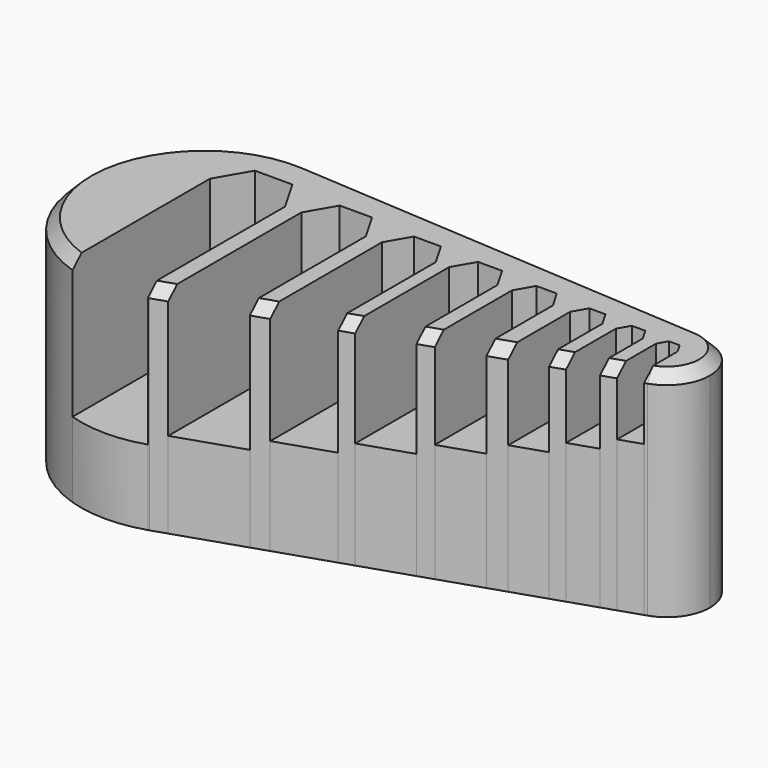
from build123d import *

# Parameters (mm, degrees)
F1_DEPTH       = 20
F2_DEPTH       = 14
F3_DEPTH       = 13
F4_DEPTH       = 12
F5_DEPTH       = 11
F6_DEPTH       = 10
F7_DEPTH       = 9
F8_DEPTH       = 8
F9_DEPTH       = 7
F10_T1_DEPTH   = 6.723420565
F10_T3_DEPTH   = 6.4600781335
F10_T5_DEPTH   = 6.5654151061
F10_T7_DEPTH   = 6.8287575376
F10_T9_DEPTH   = 6.4600781335
F10_T11_DEPTH  = 6.4600781335
F10_T13_DEPTH  = 4.0315664401
F10_T15_DEPTH  = 38.5986158262
F10_T17_DEPTH  = 2.842475063
F10_T20_ANGLE  = 178.7866538195
F10_T24_DEPTH  = 8.6433659759
F10_T30_DEPTH  = 8.6433659759
F10_T36_DEPTH  = 8.6433659759
F10_T42_DEPTH  = 8.1433659759
F10_T48_DEPTH  = 8.1433659759
F10_T54_DEPTH  = 8.1433659759
F10_T60_DEPTH  = 7.6433659759
F10_T66_DEPTH  = 7.6433659759
F10_T72_DEPTH  = 7.6433659759
F10_T78_DEPTH  = 7.3933659759
F10_T84_DEPTH  = 7.3933659759
F10_T90_DEPTH  = 7.3933659759
F10_T96_DEPTH  = 7.0433659759
F10_T102_DEPTH = 7.0433659759
F10_T108_DEPTH = 7.0433659759
F10_T114_DEPTH = 6.6433659759
F10_T120_DEPTH = 6.6433659759
F10_T126_DEPTH = 6.6433659759
F10_T130_ANGLE = 13.4104469015
F10_T132_ANGLE = 158.0080412786
F10_T137_DEPTH = 8.6433659759
F10_T141_DEPTH = 8.6433659759
F10_T149_DEPTH = 8.6433659759
F10_T153_DEPTH = 8.6433659759
F10_T161_DEPTH = 8.1433659759
F10_T166_DEPTH = 8.1433659759
F10_T173_DEPTH = 8.1433659759
F10_T177_DEPTH = 8.1433659759
F10_T185_DEPTH = 7.6433659759
F10_T190_DEPTH = 7.6433659759
F10_T197_DEPTH = 7.6433659759
F10_T201_DEPTH = 7.6433659759
F10_T209_DEPTH = 7.3933659759
F10_T214_DEPTH = 7.3933659759
F10_T221_DEPTH = 7.3933659759
F10_T226_DEPTH = 7.3933659759
F10_T233_DEPTH = 7.0433659759
F10_T238_DEPTH = 7.0433659759
F10_T246_DEPTH = 7.0433659759
F10_T251_DEPTH = 7.0433659759
F10_T259_DEPTH = 6.6433659759
F10_T264_DEPTH = 6.6433659759
F10_T272_DEPTH = 6.6433659759
F10_T277_DEPTH = 6.6433659759
F11_SIZE       = 0.5


# Not quite as in the source:
# - a fillet or chamfer that OpenCascade refuses, or shapes differently, is made with other operations: its cross-section is extruded or revolved along the edge and cut away or added


with BuildPart() as f1:
    # F0 (on Top) → F1 (new body)
    with BuildSketch(Plane.XY):
        with BuildLine():
            ThreePointArc((-17.3859174192, -15.9276489395), (-16.683828396, -15.6696039674), (-16, -15.3664622036))
            Line((-16, -15.3664622036), (-16, 0))
            Line((-16, 0), (-14.5, 2.5980762114))
            Line((-14.5, 2.5980762114), (-12.3766282, 2.5980762114))
            ThreePointArc((-12.3766282, 2.5980762114), (-15.9358837519, 5.3146518801), (-20.2628204012, 6.4660435079))
            ThreePointArc((-20.2628204012, 6.4660435079), (-32.3001541206, -2.8757046875), (-24.5, -15.9647557651))
            Line((-24.5, -15.9647557651), (-24.5, 0))
            Line((-24.5, 0), (-22.75, 3.0310889132))
            Line((-22.75, 3.0310889132), (-19.25, 3.0310889132))
            Line((-19.25, 3.0310889132), (-17.5, 0))
            Line((-17.5, 0), (-17.5, -15.9647557651))
            ThreePointArc((-17.5, -15.9647557651), (-17.4429103229, -15.9463511141), (-17.3859174192, -15.9276489395))
        make_face()
        with BuildLine():
            Line((-2.25, 0), (-1.125, 1.9485571585))
            Line((-1.125, 1.9485571585), (1.125, 1.9485571585))
            Line((1.125, 1.9485571585), (2.25, 0))
            Line((2.25, 0), (2.25, -9.4273659957))
            Line((2.25, -9.4273659957), (3.6, -8.9804613879))
            Line((3.6, -8.9804613879), (3.6, 0))
            Line((3.6, 0), (4.55, 1.6454482672))
            Line((4.55, 1.6454482672), (6.45, 1.6454482672))
            Line((6.45, 1.6454482672), (7.4, 0))
            Line((7.4, 0), (7.4, -7.7225076769))
            Line((7.4, -7.7225076769), (9, -7.1928429565))
            Line((9, -7.1928429565), (9, 0))
            Line((9, 0), (9.75, 1.2990381057))
            Line((9.75, 1.2990381057), (11.25, 1.2990381057))
            Line((11.25, 1.2990381057), (12, 0))
            Line((12, 0), (12, -6.1997216057))
            Line((12, -6.1997216057), (13.25, -5.7859210429))
            Line((13.25, -5.7859210429), (13.25, 0))
            Line((13.25, 0), (13.875, 1.0825317547))
            Line((13.875, 1.0825317547), (14.1492695498, 1.0825317547))
            ThreePointArc((14.1492695498, 1.0825317547), (15.6879217246, 3.2640916115), (18.2564102564, 3.9917732627))
            Line((18.2564102564, 3.9917732627), (-20.2628204012, 6.4660435079))
            ThreePointArc((-20.2628204012, 6.4660435079), (-15.9358837519, 5.3146518801), (-12.3766282, 2.5980762114))
            Line((-12.3766282, 2.5980762114), (-11.5, 2.5980762114))
            Line((-11.5, 2.5980762114), (-10, 0))
            Line((-10, 0), (-10, -1.6562026488))
            ThreePointArc((-10, -1.6562026488), (-9.6256868339, -3.3147221192), (-9.5, -5.010304615))
            ThreePointArc((-9.5, -5.010304615), (-9.6256868339, -6.7058871108), (-10, -8.3644065813))
            Line((-10, -8.3644065813), (-10, -13.4826115115))
            Line((-10, -13.4826115115), (-8.5, -12.9860508361))
            Line((-8.5, -12.9860508361), (-8.5, 0))
            Line((-8.5, 0), (-7.25, 2.1650635095))
            Line((-7.25, 2.1650635095), (-4.75, 2.1650635095))
            Line((-4.75, 2.1650635095), (-3.5, 0))
            Line((-3.5, 0), (-3.5, -11.3308485847))
            Line((-3.5, -11.3308485847), (-2.25, -10.9170480219))
            Line((-2.25, -10.9170480219), (-2.25, 0))
        make_face()
        with BuildLine():
            Line((15.75, 0), (15.75, -3.3071891388))
            ThreePointArc((15.75, -3.3071891388), (16.3505589519, -3.6440834552), (17, -3.8729833462))
            Line((17, -3.8729833462), (17, 0))
            Line((17, 0), (17.5, 0.8660254038))
            Line((17.5, 0.8660254038), (18.5, 0.8660254038))
            Line((18.5, 0.8660254038), (19, 0))
            Line((19, 0), (19, -3.8729833462))
            ThreePointArc((19, -3.8729833462), (19.1291697471, -3.8373136023), (19.257072202, -3.7973371563))
            ThreePointArc((19.257072202, -3.7973371563), (21.2425521436, -2.3421903415), (22, 0))
            ThreePointArc((22, 0), (20.9176738188, 2.7362710917), (18.2564102564, 3.9917732627))
            ThreePointArc((18.2564102564, 3.9917732627), (15.6879217246, 3.2640916115), (14.1492695498, 1.0825317547))
            Line((14.1492695498, 1.0825317547), (15.125, 1.0825317547))
            Line((15.125, 1.0825317547), (15.75, 0))
        make_face()
        with BuildLine():
            Line((-10, -1.6562026488), (-10, -8.3644065813))
            ThreePointArc((-10, -8.3644065813), (-9.6256868339, -6.7058871108), (-9.5, -5.010304615))
            ThreePointArc((-9.5, -5.010304615), (-9.6256868339, -3.3147221192), (-10, -1.6562026488))
        make_face()
        with BuildLine():
            Line((15.75, -3.3071891388), (15.75, -4.9583199172))
            Line((15.75, -4.9583199172), (17, -4.5445193544))
            Line((17, -4.5445193544), (17, -3.8729833462))
            ThreePointArc((17, -3.8729833462), (16.3505589519, -3.6440834552), (15.75, -3.3071891388))
        make_face()
        with BuildLine():
            Line((19, -3.8729833462), (19, -3.8824384538))
            Line((19, -3.8824384538), (19.257072202, -3.7973371563))
            ThreePointArc((19.257072202, -3.7973371563), (19.1291697471, -3.8373136023), (19, -3.8729833462))
        make_face()
        with BuildLine():
            Line((-17.3859174192, -15.9276489395), (-16, -15.468854213))
            Line((-16, -15.468854213), (-16, -15.3664622036))
            ThreePointArc((-16, -15.3664622036), (-16.683828396, -15.6696039674), (-17.3859174192, -15.9276489395))
        make_face()
    extrude(amount=F1_DEPTH)

    # F0 (on Top) → F2 (join)
    with BuildSketch(Plane.XY):
        with BuildLine():
            Line((17, 0), (17, -3.8729833462))
            ThreePointArc((17, -3.8729833462), (18, -4), (19, -3.8729833462))
            Line((19, -3.8729833462), (19, 0))
            Line((19, 0), (18.5, -0.8660254038))
            Line((18.5, -0.8660254038), (17.5, -0.8660254038))
            Line((17.5, -0.8660254038), (17, 0))
        make_face()
        with BuildLine():
            Line((17, -3.8729833462), (17, -4.5445193544))
            Line((17, -4.5445193544), (19, -3.8824384538))
            Line((19, -3.8824384538), (19, -3.8729833462))
            ThreePointArc((19, -3.8729833462), (18, -4), (17, -3.8729833462))
        make_face()
    extrude(amount=F2_DEPTH)

    # F0 (on Top) → F3 (join)
    with BuildSketch(Plane.XY):
        with BuildLine():
            Line((13.25, 0), (13.25, -5.7859210429))
            Line((13.25, -5.7859210429), (15.75, -4.9583199172))
            Line((15.75, -4.9583199172), (15.75, -3.3071891388))
            ThreePointArc((15.75, -3.3071891388), (14.7531548966, -2.3362356205), (14.1492695498, -1.0825317547))
            Line((14.1492695498, -1.0825317547), (13.875, -1.0825317547))
            Line((13.875, -1.0825317547), (13.25, 0))
        make_face()
        with BuildLine():
            ThreePointArc((14.1492695498, -1.0825317547), (14.7531548966, -2.3362356205), (15.75, -3.3071891388))
            Line((15.75, -3.3071891388), (15.75, 0))
            Line((15.75, 0), (15.125, -1.0825317547))
            Line((15.125, -1.0825317547), (14.1492695498, -1.0825317547))
        make_face()
    extrude(amount=F3_DEPTH)

    # F0 (on Top) → F4 (join)
    with BuildSketch(Plane.XY):
        Polygon((9, 0), (9, -7.1928429565), (12, -6.1997216057), (12, 0), (11.25, -1.2990381057), (9.75, -1.2990381057), align=None)
    extrude(amount=F4_DEPTH)

    # F0 (on Top) → F5 (join)
    with BuildSketch(Plane.XY):
        Polygon((3.6, 0), (3.6, -8.9804613879), (7.4, -7.7225076769), (7.4, 0), (6.45, -1.6454482672), (4.55, -1.6454482672), align=None)
    extrude(amount=F5_DEPTH)

    # F0 (on Top) → F6 (join)
    with BuildSketch(Plane.XY):
        Polygon((-1.125, -1.9485571585), (-2.25, 0), (-2.25, -10.9170480219), (2.25, -9.4273659957), (2.25, 0), (1.125, -1.9485571585), align=None)
    extrude(amount=F6_DEPTH)

    # F0 (on Top) → F7 (join)
    with BuildSketch(Plane.XY):
        Polygon((-8.5, -12.9860508361), (-3.5, -11.3308485847), (-3.5, 0), (-4.75, -2.1650635095), (-7.25, -2.1650635095), (-8.5, 0), align=None)
    extrude(amount=F7_DEPTH)

    # F0 (on Top) → F8 (join)
    with BuildSketch(Plane.XY):
        with BuildLine():
            Line((-16, -15.468854213), (-10, -13.4826115115))
            Line((-10, -13.4826115115), (-10, -8.3644065813))
            ThreePointArc((-10, -8.3644065813), (-12.2674633849, -12.4931385879), (-16, -15.3664622036))
            Line((-16, -15.3664622036), (-16, -15.468854213))
        make_face()
        with BuildLine():
            ThreePointArc((-16, -15.3664622036), (-12.2674633849, -12.4931385879), (-10, -8.3644065813))
            Line((-10, -8.3644065813), (-10, -1.6562026488))
            ThreePointArc((-10, -1.6562026488), (-10.1707020381, -1.1403814048), (-10.3655774228, -0.6331986704))
            Line((-10.3655774228, -0.6331986704), (-11.5, -2.5980762114))
            Line((-11.5, -2.5980762114), (-14.5, -2.5980762114))
            Line((-14.5, -2.5980762114), (-16, 0))
            Line((-16, 0), (-16, -15.3664622036))
        make_face()
        with BuildLine():
            ThreePointArc((-10.3655774228, -0.6331986704), (-10.1707020381, -1.1403814048), (-10, -1.6562026488))
            Line((-10, -1.6562026488), (-10, 0))
            Line((-10, 0), (-10.3655774228, -0.6331986704))
        make_face()
    extrude(amount=F8_DEPTH)

    # F0 (on Top) → F9 (join)
    with BuildSketch(Plane.XY):
        with BuildLine():
            ThreePointArc((-24.5, -15.9647557651), (-21, -16.510304615), (-17.5, -15.9647557651))
            Line((-17.5, -15.9647557651), (-17.5, 0))
            Line((-17.5, 0), (-19.25, -3.0310889132))
            Line((-19.25, -3.0310889132), (-22.75, -3.0310889132))
            Line((-22.75, -3.0310889132), (-24.5, 0))
            Line((-24.5, 0), (-24.5, -15.9647557651))
        make_face()
    extrude(amount=F9_DEPTH)

    # F10: chamfer of 1 on 29 edges, made by hand

    # F10_s2 → F10_t1 (cut)
    with BuildSketch(Plane(origin=(-15.4762183794, -5.1232543007, 0), x_dir=(0, 0, 1), z_dir=(0.9493342891, 0.3142680505, 0))):
        Polygon((20, 8.6568249091), (19, 9.6568249091), (20, 9.6568249091), align=None)
    extrude(amount=F10_T1_DEPTH, mode=Mode.SUBTRACT)

    # F10_s4 → F10_t3 (cut)
    with BuildSketch(Plane(origin=(-8.9762183794, -2.971491374, 0), x_dir=(0, 0, 1), z_dir=(0.9493342891, 0.3142680505, 0))):
        Polygon((20, 8.6568249091), (19, 9.6568249091), (20, 9.6568249091), align=None)
    extrude(amount=F10_T3_DEPTH, mode=Mode.SUBTRACT)

    # F10_s6 → F10_t5 (cut)
    with BuildSketch(Plane(origin=(-3.2262183794, -1.068008785, 0), x_dir=(0, 0, 1), z_dir=(0.9493342891, 0.3142680505, 0))):
        Polygon((20, 8.6568249091), (19, 9.6568249091), (20, 9.6568249091), align=None)
    extrude(amount=F10_T5_DEPTH, mode=Mode.SUBTRACT)

    # F10_s8 → F10_t7 (cut)
    with BuildSketch(Plane(origin=(1.9237816206, 0.6368495339, 0), x_dir=(0, 0, 1), z_dir=(0.9493342891, 0.3142680505, 0))):
        Polygon((20, 8.6568249091), (19, 9.6568249091), (20, 9.6568249091), align=None)
    extrude(amount=F10_T7_DEPTH, mode=Mode.SUBTRACT)

    # F10_s10 → F10_t9 (cut)
    with BuildSketch(Plane(origin=(6.5237816206, 2.1596356051, 0), x_dir=(0, 0, 1), z_dir=(0.9493342891, 0.3142680505, 0))):
        Polygon((20, 8.6568249091), (19, 9.6568249091), (20, 9.6568249091), align=None)
    extrude(amount=F10_T9_DEPTH, mode=Mode.SUBTRACT)

    # F10_s12 → F10_t11 (cut)
    with BuildSketch(Plane(origin=(10.2737816206, 3.4010372936, 0), x_dir=(0, 0, 1), z_dir=(0.9493342891, 0.3142680505, 0))):
        Polygon((20, 8.6568249091), (19, 9.6568249091), (20, 9.6568249091), align=None)
    extrude(amount=F10_T11_DEPTH, mode=Mode.SUBTRACT)

    # F10_s14 → F10_t13 (cut)
    with BuildSketch(Plane(origin=(-20.4207489575, -6.7600939296, 0), x_dir=(0, 0, 1), z_dir=(0.9493342891, 0.3142680505, 0))):
        Polygon((20, 8.6568249091), (19, 9.6568249091), (20, 9.6568249091), align=None)
    extrude(amount=F10_T13_DEPTH, mode=Mode.SUBTRACT)

    # F10_s16 → F10_t15 (cut)
    with BuildSketch(Plane(origin=(17.926035503, -1.1514730565, 0), x_dir=(0, 0, 1), z_dir=(-0.9979433157, 0.0641025641, 0))):
        Polygon((20, 4.1538461538), (19, 5.1538461538), (20, 5.1538461538), align=None)
    extrude(amount=F10_T15_DEPTH, mode=Mode.SUBTRACT)

    # F10_s18 → F10_t17 (cut)
    with BuildSketch(Plane(origin=(13.5237816206, 4.4769187569, 0), x_dir=(0, 0, 1), z_dir=(0.9493342891, 0.3142680505, 0))):
        Polygon((20, 8.6568249091), (19, 9.6568249091), (20, 9.6568249091), align=None)
    extrude(amount=F10_T17_DEPTH, mode=Mode.SUBTRACT)

    # F10_s19 → F10_t20 (revolve, cut)
    with BuildSketch(Plane(origin=(-20.5931951918, 1.3227973923, 0), x_dir=(0, 0, 1), z_dir=(0.997943315, -0.0641025738, 0))):
        Polygon((20, -4.1538459531), (19, -5.1538459533), (20, -5.1538459531), align=None)
    revolve(axis=Axis((-21, -5.010304615, 20), (0, 0, 1)), revolution_arc=F10_T20_ANGLE, mode=Mode.SUBTRACT)


with BuildPart() as f10_tool22:
    # F10_s23 → F10_t24 (new body)
    with BuildSketch(Plane.YZ.offset(-16.678317012)):
        Polygon((-4.0310889132, 7), (-3.0310889132, 6), (-3.0310889132, 7), align=None)
    extrude(amount=-F10_T24_DEPTH)

    split(bisect_by=Plane(origin=(-18.375, -10.6088111964, 0), x_dir=(0, 0, 1), z_dir=(0.8660254038, 0.5, 0)), keep=Keep.TOP)

    split(bisect_by=Plane(origin=(-13.125, 7.5777222831, 0), x_dir=(0, 0, 1), z_dir=(-0.8660254038, 0.5, 0)), keep=Keep.TOP)


with BuildPart() as f1_1:
    add(f1.part)

    # F10_t21: cut F10_tool22
    add(f10_tool22.part, mode=Mode.SUBTRACT)


with BuildPart() as f10_tool28:
    # F10_s29 → F10_t30 (new body)
    with BuildSketch(Plane(origin=(-3.089158506, 5.3505794851, 0), x_dir=(0, 0, 1), z_dir=(-0.5, 0.8660254038, 0))):
        Polygon((6, -21.2176223927), (7, -22.2176223927), (7, -21.2176223927), align=None)
    extrude(amount=F10_T30_DEPTH)

    split(bisect_by=Plane.XZ.offset(3.0310889132), keep=Keep.BOTTOM)

    split(bisect_by=Plane.YZ.offset(-24.5), keep=Keep.TOP)


with BuildPart() as f1_2:
    add(f1_1.part)

    # F10_t27: cut F10_tool28
    add(f10_tool28.part, mode=Mode.SUBTRACT)


with BuildPart() as f10_tool34:
    # F10_s35 → F10_t36 (new body)
    with BuildSketch(Plane(origin=(-3.089158506, -5.3505794851, 0), x_dir=(0, 0, 1), z_dir=(-0.5, -0.8660254038, 0))):
        Polygon((7, 14.1554445662), (6, 15.1554445662), (7, 15.1554445662), align=None)
    extrude(amount=F10_T36_DEPTH)

    split(bisect_by=Plane.XZ.offset(3.0310889132), keep=Keep.BOTTOM)

    split(bisect_by=Plane.YZ.offset(-17.5), keep=Keep.BOTTOM)


with BuildPart() as f1_3:
    add(f1_2.part)

    # F10_t33: cut F10_tool34
    add(f10_tool34.part, mode=Mode.SUBTRACT)


with BuildPart() as f10_tool40:
    # F10_s41 → F10_t42 (new body)
    with BuildSketch(Plane(origin=(-1.214158506, 2.1029842209, 0), x_dir=(0, 0, 1), z_dir=(-0.5, 0.8660254038, 0))):
        Polygon((8, -14.8564064606), (7, -13.8564064606), (8, -13.8564064606), align=None)
    extrude(amount=F10_T42_DEPTH)

    split(bisect_by=Plane.XZ.offset(2.5980762114), keep=Keep.BOTTOM)

    split(bisect_by=Plane.YZ.offset(-16), keep=Keep.TOP)


with BuildPart() as f1_4:
    add(f1_3.part)

    # F10_t39: cut F10_tool40
    add(f10_tool40.part, mode=Mode.SUBTRACT)


with BuildPart() as f10_tool46:
    # F10_s47 → F10_t48 (new body)
    with BuildSketch(Plane.YZ.offset(-8.928317012)):
        Polygon((-3.5980762114, 8), (-2.5980762114, 7), (-2.5980762114, 8), align=None)
    extrude(amount=-F10_T48_DEPTH)

    split(bisect_by=Plane(origin=(-12, -6.9282032303, 0), x_dir=(0, 0, 1), z_dir=(0.8660254038, 0.5, 0)), keep=Keep.TOP)

    split(bisect_by=Plane(origin=(-7.5, 4.3301270189, 0), x_dir=(0, 0, 1), z_dir=(-0.8660254038, 0.5, 0)), keep=Keep.TOP)


with BuildPart() as f1_5:
    add(f1_4.part)

    # F10_t45: cut F10_tool46
    add(f10_tool46.part, mode=Mode.SUBTRACT)


with BuildPart() as f10_tool52:
    # F10_s53 → F10_t54 (new body)
    with BuildSketch(Plane(origin=(-1.214158506, -2.1029842209, 0), x_dir=(0, 0, 1), z_dir=(-0.5, -0.8660254038, 0))):
        Polygon((8, 7.6602540378), (7, 8.6602540378), (8, 8.6602540378), align=None)
    extrude(amount=F10_T54_DEPTH)

    split(bisect_by=Plane.YZ.offset(-10), keep=Keep.BOTTOM)

    split(bisect_by=Plane.XZ.offset(2.5980762114), keep=Keep.BOTTOM)


with BuildPart() as f1_6:
    add(f1_5.part)

    # F10_t51: cut F10_tool52
    add(f10_tool52.part, mode=Mode.SUBTRACT)


with BuildPart() as f10_tool58:
    # F10_s59 → F10_t60 (new body)
    with BuildSketch(Plane(origin=(0.410841494, -0.7115983414, 0), x_dir=(0, 0, 1), z_dir=(-0.5, 0.8660254038, 0))):
        Polygon((9, -8.3612159322), (8, -7.3612159322), (9, -7.3612159322), align=None)
    extrude(amount=F10_T60_DEPTH)

    split(bisect_by=Plane.XZ.offset(2.1650635095), keep=Keep.BOTTOM)

    split(bisect_by=Plane.YZ.offset(-8.5), keep=Keep.TOP)


with BuildPart() as f1_7:
    add(f1_6.part)

    # F10_t57: cut F10_tool58
    add(f10_tool58.part, mode=Mode.SUBTRACT)


with BuildPart() as f10_tool64:
    # F10_s65 → F10_t66 (new body)
    with BuildSketch(Plane.YZ.offset(-2.178317012)):
        Polygon((-3.1650635095, 9), (-2.1650635095, 8), (-2.1650635095, 9), align=None)
    extrude(amount=-F10_T66_DEPTH)

    split(bisect_by=Plane(origin=(-6.375, -3.6806079661, 0), x_dir=(0, 0, 1), z_dir=(0.8660254038, 0.5, 0)), keep=Keep.TOP)

    split(bisect_by=Plane(origin=(-2.625, 1.5155444566, 0), x_dir=(0, 0, 1), z_dir=(-0.8660254038, 0.5, 0)), keep=Keep.TOP)


with BuildPart() as f1_8:
    add(f1_7.part)

    # F10_t63: cut F10_tool64
    add(f10_tool64.part, mode=Mode.SUBTRACT)


with BuildPart() as f10_tool70:
    # F10_s71 → F10_t72 (new body)
    with BuildSketch(Plane(origin=(0.410841494, 0.7115983414, 0), x_dir=(0, 0, 1), z_dir=(-0.5, -0.8660254038, 0))):
        Polygon((9, 2.0310889132), (8, 3.0310889132), (9, 3.0310889132), align=None)
    extrude(amount=F10_T72_DEPTH)

    split(bisect_by=Plane.YZ.offset(-3.5), keep=Keep.BOTTOM)

    split(bisect_by=Plane.XZ.offset(2.1650635095), keep=Keep.BOTTOM)


with BuildPart() as f1_9:
    add(f1_8.part)

    # F10_t69: cut F10_tool70
    add(f10_tool70.part, mode=Mode.SUBTRACT)


with BuildPart() as f10_tool76:
    # F10_s77 → F10_t78 (new body)
    with BuildSketch(Plane(origin=(1.848341494, -3.2014213773, 0), x_dir=(0, 0, 1), z_dir=(-0.5, 0.8660254038, 0))):
        Polygon((10, -2.9485571585), (9, -1.9485571585), (10, -1.9485571585), align=None)
    extrude(amount=F10_T78_DEPTH)

    split(bisect_by=Plane.XZ.offset(1.9485571585), keep=Keep.BOTTOM)

    split(bisect_by=Plane.YZ.offset(-2.25), keep=Keep.TOP)


with BuildPart() as f1_10:
    add(f1_9.part)

    # F10_t75: cut F10_tool76
    add(f10_tool76.part, mode=Mode.SUBTRACT)


with BuildPart() as f10_tool82:
    # F10_s83 → F10_t84 (new body)
    with BuildSketch(Plane.YZ.offset(3.696682988)):
        Polygon((-2.9485571585, 10), (-1.9485571585, 9), (-1.9485571585, 10), align=None)
    extrude(amount=-F10_T84_DEPTH)

    split(bisect_by=Plane(origin=(1.6875, -0.9742785793, 0), x_dir=(0, 0, 1), z_dir=(-0.8660254038, 0.5, 0)), keep=Keep.TOP)

    split(bisect_by=Plane(origin=(-1.6875, -0.9742785793, 0), x_dir=(0, 0, 1), z_dir=(0.8660254038, 0.5, 0)), keep=Keep.TOP)


with BuildPart() as f1_11:
    add(f1_10.part)

    # F10_t81: cut F10_tool82
    add(f10_tool82.part, mode=Mode.SUBTRACT)


with BuildPart() as f10_tool88:
    # F10_s89 → F10_t90 (new body)
    with BuildSketch(Plane(origin=(1.848341494, 3.2014213773, 0), x_dir=(0, 0, 1), z_dir=(-0.5, -0.8660254038, 0))):
        Polygon((10, -2.9485571585), (9, -1.9485571585), (10, -1.9485571585), align=None)
    extrude(amount=F10_T90_DEPTH)

    split(bisect_by=Plane.YZ.offset(2.25), keep=Keep.BOTTOM)

    split(bisect_by=Plane.XZ.offset(1.9485571585), keep=Keep.BOTTOM)


with BuildPart() as f1_12:
    add(f1_11.part)

    # F10_t87: cut F10_tool88
    add(f10_tool88.part, mode=Mode.SUBTRACT)


with BuildPart() as f10_tool94:
    # F10_s95 → F10_t96 (new body)
    with BuildSketch(Plane(origin=(3.135841494, -5.4314367921, 0), x_dir=(0, 0, 1), z_dir=(-0.5, 0.8660254038, 0))):
        Polygon((11, 2.1176914536), (10, 3.1176914536), (11, 3.1176914536), align=None)
    extrude(amount=F10_T96_DEPTH)

    split(bisect_by=Plane.XZ.offset(1.6454482672), keep=Keep.BOTTOM)

    split(bisect_by=Plane.YZ.offset(3.6), keep=Keep.TOP)


with BuildPart() as f1_13:
    add(f1_12.part)

    # F10_t93: cut F10_tool94
    add(f10_tool94.part, mode=Mode.SUBTRACT)


with BuildPart() as f10_tool100:
    # F10_s101 → F10_t102 (new body)
    with BuildSketch(Plane.YZ.offset(9.021682988)):
        Polygon((-2.6454482672, 11), (-1.6454482672, 10), (-1.6454482672, 11), align=None)
    extrude(amount=-F10_T102_DEPTH)

    split(bisect_by=Plane(origin=(5.55, -3.204293994, 0), x_dir=(0, 0, 1), z_dir=(-0.8660254038, 0.5, 0)), keep=Keep.TOP)

    split(bisect_by=Plane(origin=(2.7, 1.5588457268, 0), x_dir=(0, 0, 1), z_dir=(0.8660254038, 0.5, 0)), keep=Keep.TOP)


with BuildPart() as f1_14:
    add(f1_13.part)

    # F10_t99: cut F10_tool100
    add(f10_tool100.part, mode=Mode.SUBTRACT)


with BuildPart() as f10_tool106:
    # F10_s107 → F10_t108 (new body)
    with BuildSketch(Plane(origin=(3.135841494, 5.4314367921, 0), x_dir=(0, 0, 1), z_dir=(-0.5, -0.8660254038, 0))):
        Polygon((11, -7.408587988), (10, -6.408587988), (11, -6.408587988), align=None)
    extrude(amount=F10_T108_DEPTH)

    split(bisect_by=Plane.YZ.offset(7.4), keep=Keep.BOTTOM)

    split(bisect_by=Plane.XZ.offset(1.6454482672), keep=Keep.BOTTOM)


with BuildPart() as f1_15:
    add(f1_14.part)

    # F10_t105: cut F10_tool106
    add(f10_tool106.part, mode=Mode.SUBTRACT)


with BuildPart() as f10_tool112:
    # F10_s113 → F10_t114 (new body)
    with BuildSketch(Plane(origin=(4.285841494, -7.4232952208, 0), x_dir=(0, 0, 1), z_dir=(-0.5, 0.8660254038, 0))):
        Polygon((12, 6.7942286341), (11, 7.7942286341), (12, 7.7942286341), align=None)
    extrude(amount=F10_T114_DEPTH)

    split(bisect_by=Plane.XZ.offset(1.2990381057), keep=Keep.BOTTOM)

    split(bisect_by=Plane.YZ.offset(9), keep=Keep.TOP)


with BuildPart() as f1_16:
    add(f1_15.part)

    # F10_t111: cut F10_tool112
    add(f10_tool112.part, mode=Mode.SUBTRACT)


with BuildPart() as f10_tool118:
    # F10_s119 → F10_t120 (new body)
    with BuildSketch(Plane.YZ.offset(13.821682988)):
        Polygon((-2.2990381057, 12), (-1.2990381057, 11), (-1.2990381057, 12), align=None)
    extrude(amount=-F10_T120_DEPTH)

    split(bisect_by=Plane(origin=(9, -5.1961524227, 0), x_dir=(0, 0, 1), z_dir=(-0.8660254038, 0.5, 0)), keep=Keep.TOP)

    split(bisect_by=Plane(origin=(6.75, 3.897114317, 0), x_dir=(0, 0, 1), z_dir=(0.8660254038, 0.5, 0)), keep=Keep.TOP)


with BuildPart() as f1_17:
    add(f1_16.part)

    # F10_t117: cut F10_tool118
    add(f10_tool118.part, mode=Mode.SUBTRACT)


with BuildPart() as f10_tool124:
    # F10_s125 → F10_t126 (new body)
    with BuildSketch(Plane(origin=(4.285841494, 7.4232952208, 0), x_dir=(0, 0, 1), z_dir=(-0.5, -0.8660254038, 0))):
        Polygon((12, -11.3923048454), (11, -10.3923048454), (12, -10.3923048454), align=None)
    extrude(amount=F10_T126_DEPTH)

    split(bisect_by=Plane.YZ.offset(12), keep=Keep.BOTTOM)

    split(bisect_by=Plane.XZ.offset(1.2990381057), keep=Keep.BOTTOM)


with BuildPart() as f1_18:
    add(f1_17.part)

    # F10_t123: cut F10_tool124
    add(f10_tool124.part, mode=Mode.SUBTRACT)

    # F10_s129 → F10_t130 (revolve, cut)
    with BuildSketch(Plane(origin=(-21.2733305247, -1.8260812573, 0), x_dir=(0, 0, 1), z_dir=(-0.9963360691, -0.0855244843, 0))):
        Polygon((20, -13.6959330356), (19, -14.6959330356), (20, -14.6959330356), align=None)
    revolve(axis=Axis((-21.0000000001, -5.0103046148, 20), (0, 0, 1)), revolution_arc=F10_T130_ANGLE, mode=Mode.SUBTRACT)

    # F10_s131 → F10_t132 (revolve, cut)
    with BuildSketch(Plane(origin=(16.2222406637, 5.3702178536, 0), x_dir=(0, 0, 1), z_dir=(-0.9493342891, -0.3142680505, 0))):
        Polygon((20, -8.6568249091), (19, -9.6568249091), (20, -9.6568249091), align=None)
    revolve(axis=Axis((18, 0, 20), (0, 0, 1)), revolution_arc=F10_T132_ANGLE, mode=Mode.SUBTRACT)


with BuildPart() as f10_tool135:
    # F10_s136 → F10_t137 (new body)
    with BuildSketch(Plane(origin=(-3.089158506, -5.3505794851, 0), x_dir=(0, 0, 1), z_dir=(-0.5, -0.8660254038, 0))):
        Polygon((7, 14.1554445662), (6, 15.1554445662), (7, 15.1554445662), align=None)
    extrude(amount=F10_T137_DEPTH)

    split(bisect_by=Plane.XZ.offset(3.0310889132), keep=Keep.TOP)


with BuildPart() as f10_tool139:
    # F10_s140 → F10_t141 (new body)
    with BuildSketch(Plane.YZ.offset(-16.678317012)):
        Polygon((-4.0310889132, 7), (-3.0310889132, 6), (-3.0310889132, 7), align=None)
    extrude(amount=-F10_T141_DEPTH)

    split(bisect_by=Plane.YZ.offset(-17.5), keep=Keep.BOTTOM)

    split(bisect_by=Plane(origin=(-13.125, 7.5777222831, 0), x_dir=(0, 0, 1), z_dir=(0.8660254038, -0.5, 0)), keep=Keep.TOP)


with BuildPart() as f10_tool135_1:
    add(f10_tool135.part)

    # F10_t144: intersect F10_tool139
    add(f10_tool139.part, mode=Mode.INTERSECT)


with BuildPart() as f1_19:
    add(f1_18.part)

    # F10_t133: cut F10_tool135
    add(f10_tool135_1.part, mode=Mode.SUBTRACT)


with BuildPart() as f10_tool147:
    # F10_s148 → F10_t149 (new body)
    with BuildSketch(Plane(origin=(-3.089158506, 5.3505794851, 0), x_dir=(0, 0, 1), z_dir=(-0.5, 0.8660254038, 0))):
        Polygon((6, -21.2176223927), (7, -22.2176223927), (7, -21.2176223927), align=None)
    extrude(amount=F10_T149_DEPTH)

    split(bisect_by=Plane.XZ.offset(3.0310889132), keep=Keep.TOP)


with BuildPart() as f10_tool151:
    # F10_s152 → F10_t153 (new body)
    with BuildSketch(Plane.YZ.offset(-16.678317012)):
        Polygon((-4.0310889132, 7), (-3.0310889132, 6), (-3.0310889132, 7), align=None)
    extrude(amount=-F10_T153_DEPTH)

    split(bisect_by=Plane(origin=(-18.375, -10.6088111964, 0), x_dir=(0, 0, 1), z_dir=(-0.8660254038, -0.5, 0)), keep=Keep.TOP)

    split(bisect_by=Plane.YZ.offset(-24.5), keep=Keep.TOP)


with BuildPart() as f10_tool147_1:
    add(f10_tool147.part)

    # F10_t156: intersect F10_tool151
    add(f10_tool151.part, mode=Mode.INTERSECT)


with BuildPart() as f1_20:
    add(f1_19.part)

    # F10_t145: cut F10_tool147
    add(f10_tool147_1.part, mode=Mode.SUBTRACT)


with BuildPart() as f10_tool159:
    # F10_s160 → F10_t161 (new body)
    with BuildSketch(Plane.YZ.offset(-8.928317012)):
        Polygon((-3.5980762114, 8), (-2.5980762114, 7), (-2.5980762114, 8), align=None)
    extrude(amount=-F10_T161_DEPTH)

    split(bisect_by=Plane(origin=(-12, -6.9282032303, 0), x_dir=(0, 0, 1), z_dir=(-0.8660254038, -0.5, 0)), keep=Keep.TOP)

    split(bisect_by=Plane.YZ.offset(-16), keep=Keep.TOP)


with BuildPart() as f10_tool164:
    # F10_s165 → F10_t166 (new body)
    with BuildSketch(Plane(origin=(-1.214158506, 2.1029842209, 0), x_dir=(0, 0, 1), z_dir=(-0.5, 0.8660254038, 0))):
        Polygon((8, -14.8564064606), (7, -13.8564064606), (8, -13.8564064606), align=None)
    extrude(amount=F10_T166_DEPTH)

    split(bisect_by=Plane.XZ.offset(2.5980762114), keep=Keep.TOP)


with BuildPart() as f10_tool159_1:
    add(f10_tool159.part)

    # F10_t168: intersect F10_tool164
    add(f10_tool164.part, mode=Mode.INTERSECT)


with BuildPart() as f1_21:
    add(f1_20.part)

    # F10_t157: cut F10_tool159
    add(f10_tool159_1.part, mode=Mode.SUBTRACT)


with BuildPart() as f10_tool171:
    # F10_s172 → F10_t173 (new body)
    with BuildSketch(Plane(origin=(-1.214158506, -2.1029842209, 0), x_dir=(0, 0, 1), z_dir=(-0.5, -0.8660254038, 0))):
        Polygon((8, 7.6602540378), (7, 8.6602540378), (8, 8.6602540378), align=None)
    extrude(amount=F10_T173_DEPTH)

    split(bisect_by=Plane.XZ.offset(2.5980762114), keep=Keep.TOP)


with BuildPart() as f10_tool175:
    # F10_s176 → F10_t177 (new body)
    with BuildSketch(Plane.YZ.offset(-8.928317012)):
        Polygon((-3.5980762114, 8), (-2.5980762114, 7), (-2.5980762114, 8), align=None)
    extrude(amount=-F10_T177_DEPTH)

    split(bisect_by=Plane.YZ.offset(-10), keep=Keep.BOTTOM)

    split(bisect_by=Plane(origin=(-7.5, 4.3301270189, 0), x_dir=(0, 0, 1), z_dir=(0.8660254038, -0.5, 0)), keep=Keep.TOP)


with BuildPart() as f10_tool171_1:
    add(f10_tool171.part)

    # F10_t180: intersect F10_tool175
    add(f10_tool175.part, mode=Mode.INTERSECT)


with BuildPart() as f1_22:
    add(f1_21.part)

    # F10_t169: cut F10_tool171
    add(f10_tool171_1.part, mode=Mode.SUBTRACT)


with BuildPart() as f10_tool183:
    # F10_s184 → F10_t185 (new body)
    with BuildSketch(Plane.YZ.offset(-2.178317012)):
        Polygon((-3.1650635095, 9), (-2.1650635095, 8), (-2.1650635095, 9), align=None)
    extrude(amount=-F10_T185_DEPTH)

    split(bisect_by=Plane(origin=(-6.375, -3.6806079661, 0), x_dir=(0, 0, 1), z_dir=(-0.8660254038, -0.5, 0)), keep=Keep.TOP)

    split(bisect_by=Plane.YZ.offset(-8.5), keep=Keep.TOP)


with BuildPart() as f10_tool188:
    # F10_s189 → F10_t190 (new body)
    with BuildSketch(Plane(origin=(0.410841494, -0.7115983414, 0), x_dir=(0, 0, 1), z_dir=(-0.5, 0.8660254038, 0))):
        Polygon((9, -8.3612159322), (8, -7.3612159322), (9, -7.3612159322), align=None)
    extrude(amount=F10_T190_DEPTH)

    split(bisect_by=Plane.XZ.offset(2.1650635095), keep=Keep.TOP)


with BuildPart() as f10_tool183_1:
    add(f10_tool183.part)

    # F10_t192: intersect F10_tool188
    add(f10_tool188.part, mode=Mode.INTERSECT)


with BuildPart() as f1_23:
    add(f1_22.part)

    # F10_t181: cut F10_tool183
    add(f10_tool183_1.part, mode=Mode.SUBTRACT)


with BuildPart() as f10_tool195:
    # F10_s196 → F10_t197 (new body)
    with BuildSketch(Plane(origin=(0.410841494, 0.7115983414, 0), x_dir=(0, 0, 1), z_dir=(-0.5, -0.8660254038, 0))):
        Polygon((9, 2.0310889132), (8, 3.0310889132), (9, 3.0310889132), align=None)
    extrude(amount=F10_T197_DEPTH)

    split(bisect_by=Plane.XZ.offset(2.1650635095), keep=Keep.TOP)


with BuildPart() as f10_tool199:
    # F10_s200 → F10_t201 (new body)
    with BuildSketch(Plane.YZ.offset(-2.178317012)):
        Polygon((-3.1650635095, 9), (-2.1650635095, 8), (-2.1650635095, 9), align=None)
    extrude(amount=-F10_T201_DEPTH)

    split(bisect_by=Plane.YZ.offset(-3.5), keep=Keep.BOTTOM)

    split(bisect_by=Plane(origin=(-2.625, 1.5155444566, 0), x_dir=(0, 0, 1), z_dir=(0.8660254038, -0.5, 0)), keep=Keep.TOP)


with BuildPart() as f10_tool195_1:
    add(f10_tool195.part)

    # F10_t204: intersect F10_tool199
    add(f10_tool199.part, mode=Mode.INTERSECT)


with BuildPart() as f1_24:
    add(f1_23.part)

    # F10_t193: cut F10_tool195
    add(f10_tool195_1.part, mode=Mode.SUBTRACT)


with BuildPart() as f10_tool207:
    # F10_s208 → F10_t209 (new body)
    with BuildSketch(Plane.YZ.offset(3.696682988)):
        Polygon((-2.9485571585, 10), (-1.9485571585, 9), (-1.9485571585, 10), align=None)
    extrude(amount=-F10_T209_DEPTH)

    split(bisect_by=Plane(origin=(-1.6875, -0.9742785793, 0), x_dir=(0, 0, 1), z_dir=(-0.8660254038, -0.5, 0)), keep=Keep.TOP)

    split(bisect_by=Plane.YZ.offset(-2.25), keep=Keep.TOP)


with BuildPart() as f10_tool212:
    # F10_s213 → F10_t214 (new body)
    with BuildSketch(Plane(origin=(1.848341494, -3.2014213773, 0), x_dir=(0, 0, 1), z_dir=(-0.5, 0.8660254038, 0))):
        Polygon((10, -2.9485571585), (9, -1.9485571585), (10, -1.9485571585), align=None)
    extrude(amount=F10_T214_DEPTH)

    split(bisect_by=Plane.XZ.offset(1.9485571585), keep=Keep.TOP)


with BuildPart() as f10_tool207_1:
    add(f10_tool207.part)

    # F10_t216: intersect F10_tool212
    add(f10_tool212.part, mode=Mode.INTERSECT)


with BuildPart() as f1_25:
    add(f1_24.part)

    # F10_t205: cut F10_tool207
    add(f10_tool207_1.part, mode=Mode.SUBTRACT)


with BuildPart() as f10_tool219:
    # F10_s220 → F10_t221 (new body)
    with BuildSketch(Plane.YZ.offset(3.696682988)):
        Polygon((-2.9485571585, 10), (-1.9485571585, 9), (-1.9485571585, 10), align=None)
    extrude(amount=-F10_T221_DEPTH)

    split(bisect_by=Plane.YZ.offset(2.25), keep=Keep.BOTTOM)

    split(bisect_by=Plane(origin=(1.6875, -0.9742785793, 0), x_dir=(0, 0, 1), z_dir=(0.8660254038, -0.5, 0)), keep=Keep.TOP)


with BuildPart() as f10_tool224:
    # F10_s225 → F10_t226 (new body)
    with BuildSketch(Plane(origin=(1.848341494, 3.2014213773, 0), x_dir=(0, 0, 1), z_dir=(-0.5, -0.8660254038, 0))):
        Polygon((10, -2.9485571585), (9, -1.9485571585), (10, -1.9485571585), align=None)
    extrude(amount=F10_T226_DEPTH)

    split(bisect_by=Plane.XZ.offset(1.9485571585), keep=Keep.TOP)


with BuildPart() as f10_tool219_1:
    add(f10_tool219.part)

    # F10_t228: intersect F10_tool224
    add(f10_tool224.part, mode=Mode.INTERSECT)


with BuildPart() as f1_26:
    add(f1_25.part)

    # F10_t217: cut F10_tool219
    add(f10_tool219_1.part, mode=Mode.SUBTRACT)


with BuildPart() as f10_tool231:
    # F10_s232 → F10_t233 (new body)
    with BuildSketch(Plane.YZ.offset(9.021682988)):
        Polygon((-2.6454482672, 11), (-1.6454482672, 10), (-1.6454482672, 11), align=None)
    extrude(amount=-F10_T233_DEPTH)

    split(bisect_by=Plane(origin=(2.7, 1.5588457268, 0), x_dir=(0, 0, 1), z_dir=(-0.8660254038, -0.5, 0)), keep=Keep.TOP)

    split(bisect_by=Plane.YZ.offset(3.6), keep=Keep.TOP)


with BuildPart() as f10_tool236:
    # F10_s237 → F10_t238 (new body)
    with BuildSketch(Plane(origin=(3.135841494, -5.4314367921, 0), x_dir=(0, 0, 1), z_dir=(-0.5, 0.8660254038, 0))):
        Polygon((11, 2.1176914536), (10, 3.1176914536), (11, 3.1176914536), align=None)
    extrude(amount=F10_T238_DEPTH)

    split(bisect_by=Plane.XZ.offset(1.6454482672), keep=Keep.TOP)

    split(bisect_by=Plane.YZ.offset(3.6), keep=Keep.TOP)


with BuildPart() as f10_tool231_1:
    add(f10_tool231.part)

    # F10_t241: intersect F10_tool236
    add(f10_tool236.part, mode=Mode.INTERSECT)


with BuildPart() as f1_27:
    add(f1_26.part)

    # F10_t229: cut F10_tool231
    add(f10_tool231_1.part, mode=Mode.SUBTRACT)


with BuildPart() as f10_tool244:
    # F10_s245 → F10_t246 (new body)
    with BuildSketch(Plane.YZ.offset(9.021682988)):
        Polygon((-2.6454482672, 11), (-1.6454482672, 10), (-1.6454482672, 11), align=None)
    extrude(amount=-F10_T246_DEPTH)

    split(bisect_by=Plane.YZ.offset(7.4), keep=Keep.BOTTOM)

    split(bisect_by=Plane(origin=(5.55, -3.204293994, 0), x_dir=(0, 0, 1), z_dir=(0.8660254038, -0.5, 0)), keep=Keep.TOP)


with BuildPart() as f10_tool249:
    # F10_s250 → F10_t251 (new body)
    with BuildSketch(Plane(origin=(3.135841494, 5.4314367921, 0), x_dir=(0, 0, 1), z_dir=(-0.5, -0.8660254038, 0))):
        Polygon((11, -7.408587988), (10, -6.408587988), (11, -6.408587988), align=None)
    extrude(amount=F10_T251_DEPTH)

    split(bisect_by=Plane.YZ.offset(7.4), keep=Keep.BOTTOM)

    split(bisect_by=Plane.XZ.offset(1.6454482672), keep=Keep.TOP)


with BuildPart() as f10_tool244_1:
    add(f10_tool244.part)

    # F10_t254: intersect F10_tool249
    add(f10_tool249.part, mode=Mode.INTERSECT)


with BuildPart() as f1_28:
    add(f1_27.part)

    # F10_t242: cut F10_tool244
    add(f10_tool244_1.part, mode=Mode.SUBTRACT)


with BuildPart() as f10_tool257:
    # F10_s258 → F10_t259 (new body)
    with BuildSketch(Plane(origin=(4.285841494, -7.4232952208, 0), x_dir=(0, 0, 1), z_dir=(-0.5, 0.8660254038, 0))):
        Polygon((12, 6.7942286341), (11, 7.7942286341), (12, 7.7942286341), align=None)
    extrude(amount=F10_T259_DEPTH)

    split(bisect_by=Plane.XZ.offset(1.2990381057), keep=Keep.TOP)

    split(bisect_by=Plane.YZ.offset(9), keep=Keep.TOP)


with BuildPart() as f10_tool262:
    # F10_s263 → F10_t264 (new body)
    with BuildSketch(Plane.YZ.offset(13.821682988)):
        Polygon((-2.2990381057, 12), (-1.2990381057, 11), (-1.2990381057, 12), align=None)
    extrude(amount=-F10_T264_DEPTH)

    split(bisect_by=Plane(origin=(6.75, 3.897114317, 0), x_dir=(0, 0, 1), z_dir=(-0.8660254038, -0.5, 0)), keep=Keep.TOP)

    split(bisect_by=Plane.YZ.offset(9), keep=Keep.TOP)


with BuildPart() as f10_tool257_1:
    add(f10_tool257.part)

    # F10_t267: intersect F10_tool262
    add(f10_tool262.part, mode=Mode.INTERSECT)


with BuildPart() as f1_29:
    add(f1_28.part)

    # F10_t255: cut F10_tool257
    add(f10_tool257_1.part, mode=Mode.SUBTRACT)


with BuildPart() as f10_tool270:
    # F10_s271 → F10_t272 (new body)
    with BuildSketch(Plane(origin=(4.285841494, 7.4232952208, 0), x_dir=(0, 0, 1), z_dir=(-0.5, -0.8660254038, 0))):
        Polygon((12, -11.3923048454), (11, -10.3923048454), (12, -10.3923048454), align=None)
    extrude(amount=F10_T272_DEPTH)

    split(bisect_by=Plane.YZ.offset(12), keep=Keep.BOTTOM)

    split(bisect_by=Plane.XZ.offset(1.2990381057), keep=Keep.TOP)


with BuildPart() as f10_tool275:
    # F10_s276 → F10_t277 (new body)
    with BuildSketch(Plane.YZ.offset(13.821682988)):
        Polygon((-2.2990381057, 12), (-1.2990381057, 11), (-1.2990381057, 12), align=None)
    extrude(amount=-F10_T277_DEPTH)

    split(bisect_by=Plane.YZ.offset(12), keep=Keep.BOTTOM)

    split(bisect_by=Plane(origin=(9, -5.1961524227, 0), x_dir=(0, 0, 1), z_dir=(0.8660254038, -0.5, 0)), keep=Keep.TOP)


with BuildPart() as f10_tool270_1:
    add(f10_tool270.part)

    # F10_t280: intersect F10_tool275
    add(f10_tool275.part, mode=Mode.INTERSECT)


with BuildPart() as f1_30:
    add(f1_29.part)

    # F10_t268: cut F10_tool270
    add(f10_tool270_1.part, mode=Mode.SUBTRACT)

    # F11
    f11_edges = [f1_30.edges().sort_by_distance(p)[0] for p in [
        (13.5625, -0.541266, 13),
        (14.5, -1.082532, 13),
        (15.4375, -0.541266, 13),
        (17.25, -0.433013, 14),
        (18, -0.866025, 14),
        (18.75, -0.433013, 14),
    ]]
    chamfer(f11_edges, length=F11_SIZE)


solid = f1_30.part
